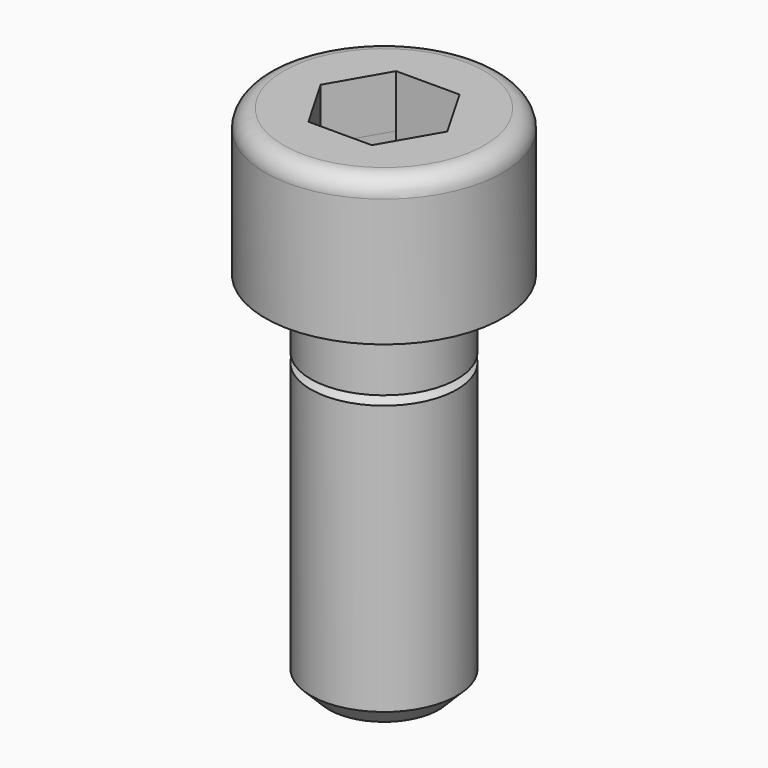
from build123d import *

# Parameters (mm, degrees)
F2_R     = 1
F3_SIZE  = 1
F5_DEPTH = 2.88


# Not quite as in the source:
# - a fillet or chamfer that OpenCascade refuses, or shapes differently, is made with other operations: its cross-section is extruded or revolved along the edge and cut away or added


with BuildPart() as f1:
    # F0 (on Front) → F1 (revolve)
    with BuildSketch(Plane.XZ):
        Polygon((-4, 0), (0, 0), (0, 21.056624327), (-2.5, 22.5), (-2.5, 28), (-6.5, 28), (-6.5, 20), (-4, 20), (-4, 16.25), (-3.5, 16), (-4, 15.75), align=None)
    revolve(axis=Axis((0, 0, 18.332445994), (0, 0, 1)))

    # F2
    f2_edges = [f1.edges().sort_by_distance(p)[0] for p in [
        (6.5, 0, 28),
    ]]
    fillet(f2_edges, radius=F2_R)

    # F3
    f3_edges = [f1.edges().sort_by_distance(p)[0] for p in [
        (4, 0, 0),
    ]]
    chamfer(f3_edges, length=F3_SIZE)

    # F4 (on face) → F5 (cut)
    with BuildSketch(Plane.XY.offset(28)):
        Polygon((-1.7320508076, -3), (1.7320508076, -3), (3.4641016151, 0), (1.7320508076, 3), (-1.7320508076, 3), (-3.4641016151, 0), align=None)
    extrude(amount=-F5_DEPTH, mode=Mode.SUBTRACT)

    # F6: chamfer of 1.5 x 2.5980762114 on 1 edges, made by hand


with BuildPart() as f6_tool2:
    # F6_s3 → F6_t4 (revolve)
    with BuildSketch(Plane.XZ):
        Polygon((-5.0980762114, 25.12), (-2.5, 23.62), (-2.5, 25.12), align=None)
    revolve(axis=Axis((0, 0, 25.12), (0, 0, 1)))

    split(bisect_by=Plane(origin=(-2.5980762114, -1.5, 0), x_dir=(0, 0, 1), z_dir=(0.8660254038, 0.5, 0)), keep=Keep.TOP)

    split(bisect_by=Plane(origin=(-2.5980762114, 1.5, 0), x_dir=(0, 0, 1), z_dir=(0.8660254038, -0.5, 0)), keep=Keep.TOP)

    split(bisect_by=Plane.XZ.offset(-3), keep=Keep.TOP)

    split(bisect_by=Plane(origin=(2.5980762114, 1.5, 0), x_dir=(0, 0, 1), z_dir=(-0.8660254038, -0.5, 0)), keep=Keep.TOP)

    split(bisect_by=Plane(origin=(2.5980762114, -1.5, 0), x_dir=(0, 0, 1), z_dir=(-0.8660254038, 0.5, 0)), keep=Keep.TOP)

    split(bisect_by=Plane.XZ.offset(3), keep=Keep.BOTTOM)


with BuildPart() as f1_1:
    add(f1.part)

    # F6_t1: cut F6_tool2
    add(f6_tool2.part, mode=Mode.SUBTRACT)


solid = f1_1.part
